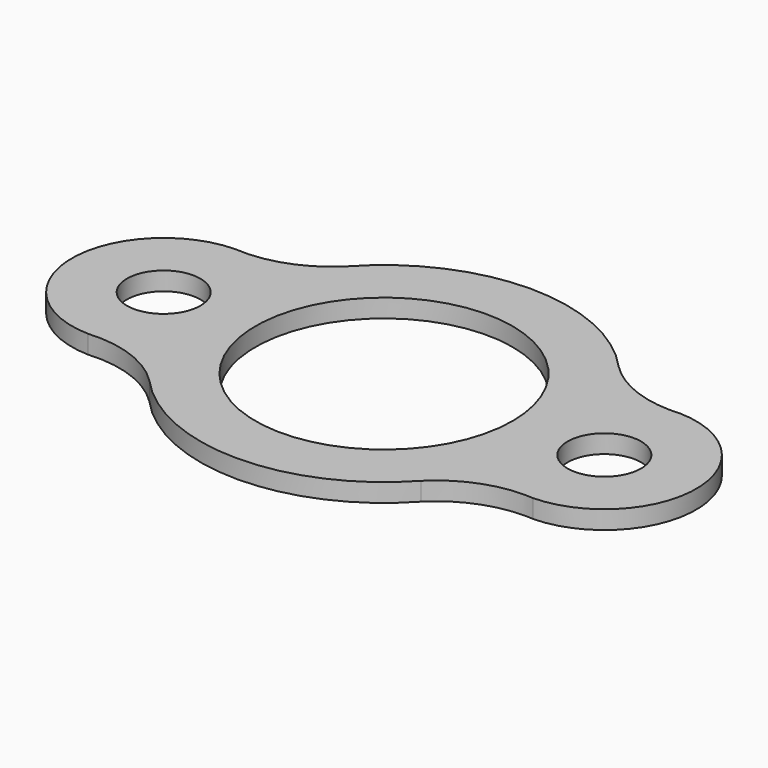
from build123d import *

# Parameters (mm, degrees)
F0_R     = 12.7
F0_R_2   = 44.45
F1_DEPTH = 3.175


# Not quite as in the source:
# - a feature names something its author has since deleted; it is built from what else it names


with BuildPart() as f1:
    # F0 (on Top) → F1 (new body, symmetric)
    with BuildSketch(Plane.XY):
        with BuildLine():
            ThreePointArc((46.9318292839, -42.7744479808), (59.0683155093, -34.6129457767), (73.3853173936, -31.624991096))
            ThreePointArc((73.3853173936, -31.624991096), (75.1406474031, -31.6432934166), (76.8932712405, -31.7424301998))
            ThreePointArc((76.8932712405, -31.7424301998), (107.95, 0), (76.8932712405, 31.7424301998))
            ThreePointArc((76.8932712405, 31.7424301998), (75.1406474031, 31.6432934166), (73.3853173936, 31.624991096))
            ThreePointArc((73.3853173936, 31.624991096), (59.0683155093, 34.6129457767), (46.9318292839, 42.7744479808))
            ThreePointArc((46.9318292839, 42.7744479808), (0, 63.5), (-46.9318292839, 42.7744479808))
            ThreePointArc((-46.9318292839, 42.7744479808), (-60.7012108245, 33.968607894), (-76.8932712405, 31.7424301998))
            ThreePointArc((-76.8932712405, 31.7424301998), (-107.95, 0), (-76.8932712405, -31.7424301998))
            ThreePointArc((-76.8932712405, -31.7424301998), (-60.7012108245, -33.968607894), (-46.9318292839, -42.7744479808))
            ThreePointArc((-46.9318292839, -42.7744479808), (0, -63.5), (46.9318292839, -42.7744479808))
        make_face()
        with Locations((-76.2, 0)):
            Circle(F0_R, mode=Mode.SUBTRACT)
        Circle(F0_R_2, mode=Mode.SUBTRACT)
        with Locations((76.2, 0)):
            Circle(F0_R, mode=Mode.SUBTRACT)
    extrude(amount=F1_DEPTH, both=True)


solid = f1.part
